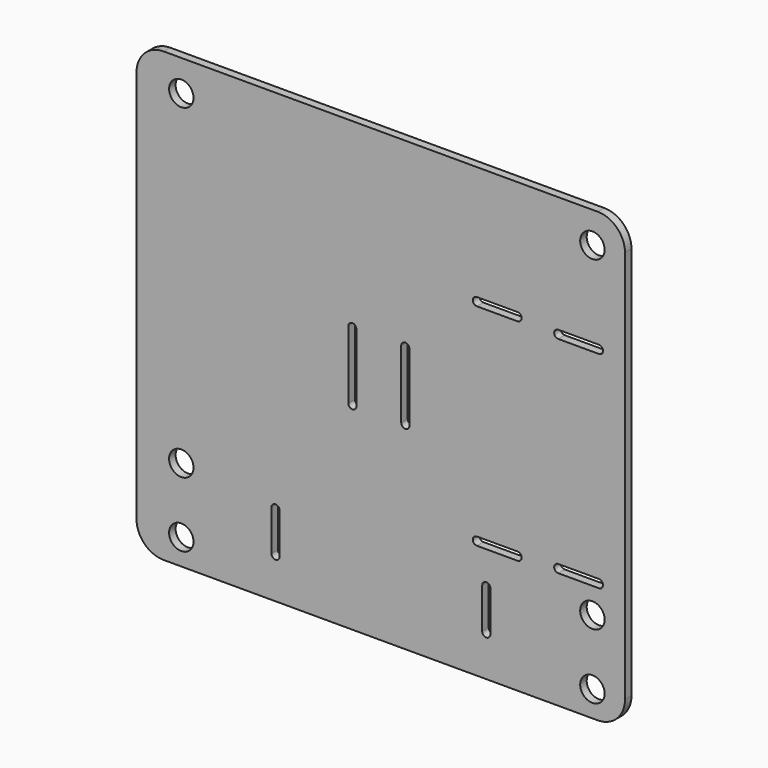
from build123d import *

# Parameters (mm, degrees)
F0_R     = 4.5
F1_DEPTH = 3


# Not quite as in the source:
# - ends of sketch curves that miss each other by under 0.0002 mm in the source are joined


with BuildPart() as f1:
    # F0 (on Front) → F1 (new body)
    with BuildSketch(Plane.XZ):
        with BuildLine():
            ThreePointArc((-123.4212349358, 88.5414632024), (-130.4923027477, 85.6125310143), (-133.4212349358, 78.5414632024))
            Line((-133.4212349358, 78.5414632024), (-133.4212349358, -66.4585367976))
            ThreePointArc((-133.4212349358, -66.4585367976), (-130.4923027477, -73.5296046095), (-123.4212349358, -76.4585367976))
            Line((-123.4212349358, -76.4585367976), (36.5787650642, -76.4585367976))
            ThreePointArc((36.5787650642, -76.4585367976), (43.6498328761, -73.5296046095), (46.5787650642, -66.4585367976))
            Line((46.5787650642, -66.4585367976), (46.5787650642, 78.5414632024))
            ThreePointArc((46.5787650642, 78.5414632024), (43.6498328761, 85.6125310143), (36.5787650642, 88.5414632024))
            Line((36.5787650642, 88.5414632024), (-123.4212349358, 88.5414632024))
        make_face()
        with Locations((-116.9212349358, -66.9585367976)):
            Circle(F0_R, mode=Mode.SUBTRACT)
        with Locations((-116.9212349358, -42.9585367976)):
            Circle(F0_R, mode=Mode.SUBTRACT)
        with BuildLine():
            Line((-80.7012349358, -46.4585367976), (-80.7012349358, -61.4585367976))
            ThreePointArc((-80.7012349358, -61.4585367976), (-82.2012349358, -62.9585367976), (-83.7012349358, -61.4585367976))
            Line((-83.7012349358, -61.4585367976), (-83.7012349358, -46.4585367976))
            ThreePointArc((-83.7012349358, -46.4585367976), (-82.2012349358, -44.9585367976), (-80.7012349358, -46.4585367976))
        make_face(mode=Mode.SUBTRACT)
        with BuildLine():
            ThreePointArc((-3.0212349358, -61.4585367976), (-4.5212349358, -62.9585367976), (-6.0212349358, -61.4585367976))
            Line((-6.0212349358, -61.4585367976), (-6.0212349358, -46.4585367976))
            ThreePointArc((-6.0212349358, -46.4585367976), (-4.5212349358, -44.9585367976), (-3.0212349358, -46.4585367976))
            Line((-3.0212349358, -46.4585367976), (-3.0212349358, -61.4585367976))
        make_face(mode=Mode.SUBTRACT)
        with Locations((34.5787650642, -66.9585362183)):
            Circle(F0_R, mode=Mode.SUBTRACT)
        with Locations((34.5787650642, -42.9585362183)):
            Circle(F0_R, mode=Mode.SUBTRACT)
        with BuildLine():
            ThreePointArc((-8, -34.2985367976), (-9.5, -32.7985367976), (-8, -31.2985367976))
            Line((-8, -31.2985367976), (7, -31.2985367976))
            ThreePointArc((7, -31.2985367976), (8.5, -32.7985367976), (7, -34.2985367976))
            Line((7, -34.2985367976), (0, -34.2985367976))
            Line((0, -34.2985367976), (-8, -34.2985367976))
        make_face(mode=Mode.SUBTRACT)
        with BuildLine():
            ThreePointArc((22, -33.4585367976), (20.5, -31.9585367976), (22, -30.4585367976))
            Line((22, -30.4585367976), (37, -30.4585367976))
            ThreePointArc((37, -30.4585367976), (38.5, -31.9585367976), (37, -33.4585367976))
            Line((37, -33.4585367976), (22, -33.4585367976))
        make_face(mode=Mode.SUBTRACT)
        with BuildLine():
            ThreePointArc((-55.3851271454, 21.5414632024), (-53.8851271454, 23.0414632024), (-52.3851271454, 21.5414632024))
            Line((-52.3851271454, 21.5414632024), (-52.3738959134, -3.4585362183))
            ThreePointArc((-52.3738959134, -3.4585362183), (-53.8738959134, -4.9585367976), (-55.3738959134, -3.4585362183))
            Line((-55.3738959134, -3.4585362183), (-55.3851271454, 21.5414632024))
        make_face(mode=Mode.SUBTRACT)
        with Locations((-116.9212349358, 77.0414632024)):
            Circle(F0_R, mode=Mode.SUBTRACT)
        with BuildLine():
            ThreePointArc((-32.8738959134, -3.4585371545), (-34.3738959134, -4.9585367976), (-35.8738959134, -3.4585371545))
            Line((-35.8738959134, -3.4585371545), (-35.8738959134, 21.5414632024))
            ThreePointArc((-35.8738959134, 21.5414632024), (-34.3738959134, 23.0414632024), (-32.8738959134, 21.5414632024))
            Line((-32.8738959134, 21.5414632024), (-32.8738959134, -3.4585371545))
        make_face(mode=Mode.SUBTRACT)
        with BuildLine():
            Line((7, 43.3814632024), (-8, 43.3814632024))
            ThreePointArc((-8, 43.3814632024), (-9.5, 44.8814632024), (-8, 46.3814632024))
            Line((-8, 46.3814632024), (7, 46.3814632024))
            ThreePointArc((7, 46.3814632024), (8.5, 44.8814632024), (7, 43.3814632024))
        make_face(mode=Mode.SUBTRACT)
        with BuildLine():
            Line((22, 45.5414632024), (37, 45.5414632024))
            ThreePointArc((37, 45.5414632024), (38.5, 44.0414632024), (37, 42.5414632024))
            Line((37, 42.5414632024), (22, 42.5414632024))
            ThreePointArc((22, 42.5414632024), (20.5, 44.0414632024), (22, 45.5414632024))
        make_face(mode=Mode.SUBTRACT)
        with Locations((34.5787650642, 77.0414632024)):
            Circle(F0_R, mode=Mode.SUBTRACT)
    extrude(amount=F1_DEPTH)


solid = f1.part
